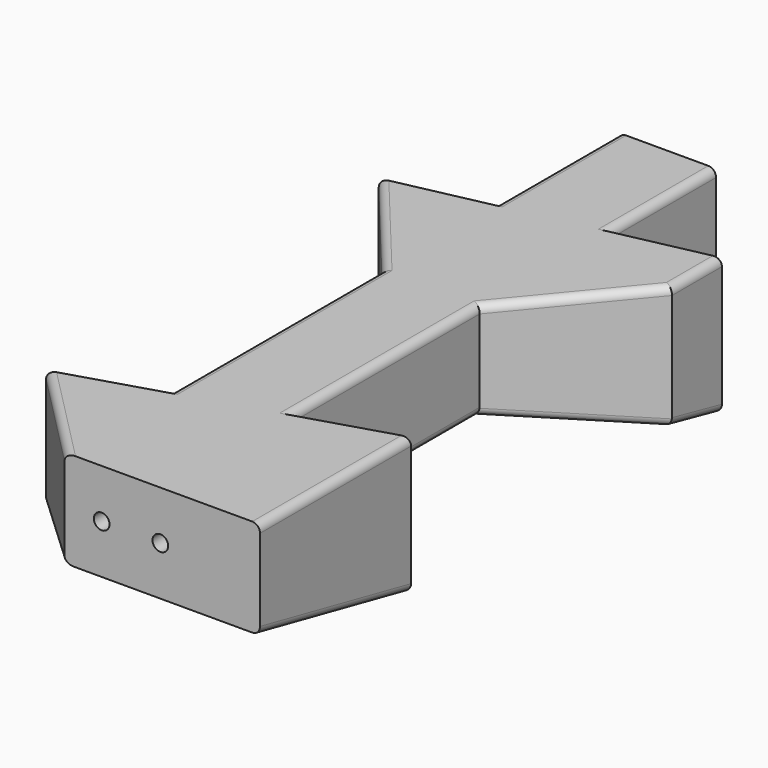
from build123d import *

# Parameters (mm, degrees)
F0_W           = 25
F0_H           = 33
F1_DEPTH       = 25
F3_DEPTH       = 10
F5_DEPTH       = 81.7
F7_DEPTH       = 10
F9_DEPTH       = 92
F10_W          = 13
F10_H          = 13
F11_DEPTH      = 135
F12_R          = 1.9
F13_DEPTH      = 7
F14_R          = 1.9
F15_DEPTH      = 7
F17_DEPTH      = 18
F18_T1_DEPTH   = 26.3114146799
F18_T3_DEPTH   = 25.9417421253
F18_T5_DEPTH   = 59.3111485648
F18_T7_DEPTH   = 58.2865340729
F18_T9_DEPTH   = 45.6084808239
F18_T11_DEPTH  = 44.6581070284
F18_T16_DEPTH  = 49.2253281189
F18_T21_DEPTH  = 48.4985768834
F18_T27_DEPTH  = 48.4985768834
F18_T33_DEPTH  = 48.4985768834
F18_T39_DEPTH  = 48.4985768834
F18_T45_DEPTH  = 48.4985768834
F18_T51_DEPTH  = 48.4985768834
F18_T57_DEPTH  = 49.2253281189
F18_T62_DEPTH  = 70.8165659944
F18_T69_DEPTH  = 70.8165659944
F18_T75_DEPTH  = 70.8165659944
F18_T81_DEPTH  = 70.8165659944
F18_T87_DEPTH  = 78.4598330308
F18_T93_DEPTH  = 78.4598330308
F18_T99_DEPTH  = 78.4598330308
F18_T106_DEPTH = 78.4598330308
F18_T112_DEPTH = 50
F18_T117_DEPTH = 50
F18_T122_DEPTH = 44.6860859582
F18_T127_DEPTH = 44.6860859582
F18_T133_DEPTH = 70.8165659944
F18_T137_DEPTH = 49.2253281189
F18_T144_DEPTH = 70.8165659944
F18_T149_DEPTH = 48.4985768834
F18_T157_DEPTH = 48.4985768834
F18_T162_DEPTH = 78.4598330308
F18_T170_DEPTH = 49.2253281189
F18_T174_DEPTH = 78.4598330308


# Not quite as in the source:
# - a fillet or chamfer that OpenCascade refuses, or shapes differently, is made with other operations: its cross-section is extruded or revolved along the edge and cut away or added


with BuildPart() as f1:
    # F0 (on Top) → F1 (new body)
    with BuildSketch(Plane.XY):
        with Locations((12.5, 16.5)):
            Rectangle(F0_W, F0_H)
        Polygon((-25, 25.3567329635), (0, 0), (0, 33), align=None)
        with Locations((37.5, 16.5)):
            Rectangle(F0_W, F0_H)
        Polygon((25, 40.6432670365), (0, 33), (25, 33), align=None)
        Polygon((0, 101.4598330308), (0, 33), (25, 40.6432670365), (25, 101.4598330308), (25, 137), (0, 137), align=None)
        Polygon((25, 40.6432670365), (25, 33), (50, 33), (50, 48.2865340729), align=None)
        Polygon((-25, 131.6860859582), (0, 101.4598330308), (0, 137), align=None)
        Polygon((25, 137), (25, 101.4598330308), (50, 131.6860859582), (50, 147.6278280835), (25, 142.3139140418), align=None)
        Polygon((25, 142.3139140418), (0, 137), (25, 137), align=None)
        Polygon((0, 177), (0, 137), (25, 142.3139140418), (25, 177), align=None)
    extrude(amount=F1_DEPTH)

    # F2 (on face) → F3 (join)
    with BuildSketch(Plane(origin=(0, 0, 0), x_dir=(1, 0, 0), z_dir=(0, 0, -1))):
        Polygon((50, -131.6860859582), (25, -101.4598330308), (0, -101.4598330308), (-25, -131.6860859582), (50, -147.6278280835), align=None)
    extrude(amount=F3_DEPTH)

    # F4 (on face) → F5 (cut, symmetric)
    with BuildSketch(Plane.YZ.offset(25)):
        Polygon((101.4598330308, -21.1370438337), (147.6278330308, -10), (101.4598330308, 0), align=None)
    extrude(amount=F5_DEPTH, both=True, mode=Mode.SUBTRACT)

    # F6 (on face) → F7 (join)
    with BuildSketch(Plane(origin=(0, 0, 0), x_dir=(1, 0, 0), z_dir=(0, 0, -1))):
        Polygon((50, -48.2865340729), (50, 0), (0, 0), (-25, -25.3567329635), align=None)
    extrude(amount=F7_DEPTH)

    # F8 (on face) → F9 (cut)
    with BuildSketch(Plane.YZ.offset(50)):
        Polygon((48.2865340729, -10), (0, 0), (0, -39.534393698), (48.2865340729, -39.534393698), align=None)
    extrude(amount=-F9_DEPTH, mode=Mode.SUBTRACT)

    # F10 (on face) → F11 (cut)
    with BuildSketch(Plane(origin=(0, 177, 0), x_dir=(-1, 0, 0), z_dir=(0, 1, 0))):
        with Locations((-12.5, 12.5)):
            Rectangle(F10_W, F10_H)
    extrude(amount=-F11_DEPTH, mode=Mode.SUBTRACT)

    # F12 (on face) → F13 (cut)
    with BuildSketch(Plane(origin=(-27.8614600507, 131.0778638485, 0), x_dir=(-0.9781476007, -0.2079116908, 0), z_dir=(-0.2079116908, 0.9781476007, 0))):
        with Locations((-18.6253867704, 12.5)):
            Circle(F12_R)
        with BuildLine():
            ThreePointArc((-72.2009313853, 12.5), (-70.3009313853, 10.6), (-68.4009313853, 12.5))
            ThreePointArc((-68.4009313853, 12.5), (-70.3009313853, 14.4), (-72.2009313853, 12.5))
        make_face()
    extrude(amount=-F13_DEPTH, mode=Mode.SUBTRACT)

    # F14 (on face) → F15 (cut)
    with BuildSketch(Plane(origin=(-9.2266829073, 30.1791199472, 0), x_dir=(-0.956304756, -0.2923717047, 0), z_dir=(-0.2923717047, 0.956304756, 0))):
        with Locations((0.6940276563, 12.5)):
            Circle(F14_R)
        with BuildLine():
            ThreePointArc((-54.6362143833, 12.2785296088), (-52.7659137894, 10.3211052927), (-50.8370889828, 12.2208866302))
            ThreePointArc((-50.8370889828, 12.2208866302), (-52.7082641762, 14.1206679678), (-54.6362143833, 12.2785296088))
        make_face()
    extrude(amount=-F15_DEPTH, mode=Mode.SUBTRACT)

    # F16 (on face) → F17 (cut)
    with BuildSketch(Plane.XZ):
        with BuildLine():
            ThreePointArc((11.5, 12.5), (9.5, 14.5), (7.5, 12.5))
            Line((7.5, 12.5), (9.5, 12.5))
            Line((9.5, 12.5), (11.5, 12.5))
        make_face()
        with BuildLine():
            ThreePointArc((26.5, 12.5), (24.5, 14.5), (22.5, 12.5))
            ThreePointArc((22.5, 12.5), (24.5, 10.5), (26.5, 12.5))
        make_face()
        with BuildLine():
            Line((9.5, 12.5), (7.5, 12.5))
            ThreePointArc((7.5, 12.5), (9.5, 10.5), (11.5, 12.5))
            Line((11.5, 12.5), (9.5, 12.5))
        make_face()
    extrude(amount=-F17_DEPTH, mode=Mode.SUBTRACT)

    # F18: fillet of radius 2 on 18 edges, made by hand

    # F18_s2 → F18_t1 (cut)
    with BuildSketch(Plane(origin=(0, 122.2526609766, -26.4799560251), x_dir=(1, 0, 0), z_dir=(0, 0.9773365731, -0.2116913388))):
        with BuildLine():
            ThreePointArc((50, -23.478167891), (49.4142135624, -22.0639543286), (48, -21.478167891))
            Line((48, -21.478167891), (50, -21.478167891))
            Line((50, -21.478167891), (50, -23.478167891))
        make_face()
    extrude(amount=F18_T1_DEPTH, mode=Mode.SUBTRACT)

    # F18_s4 → F18_t3 (cut)
    with BuildSketch(Plane.XZ.offset(-152.6278280835)):
        with BuildLine():
            ThreePointArc((48, 25), (49.4142135624, 24.4142135624), (50, 23))
            Line((50, 23), (50, 25))
            Line((50, 25), (48, 25))
        make_face()
    extrude(amount=F18_T3_DEPTH, mode=Mode.SUBTRACT)

    # F18_s6 → F18_t5 (cut)
    with BuildSketch(Plane(origin=(0, 53.1826412899, -11.0139694867), x_dir=(1, 0, 0), z_dir=(0, -0.9792214434, 0.2027938973))):
        with BuildLine():
            ThreePointArc((48, 0), (49.4142135624, 0.5857864376), (50, 2))
            Line((50, 2), (50, 0))
            Line((50, 0), (48, 0))
        make_face()
    extrude(amount=F18_T5_DEPTH, mode=Mode.SUBTRACT)

    # F18_s8 → F18_t7 (cut)
    with BuildSketch(Plane.XZ.offset(-53.2865340729)):
        with BuildLine():
            ThreePointArc((48, 25), (49.4142135624, 24.4142135624), (50, 23))
            Line((50, 23), (50, 25))
            Line((50, 25), (48, 25))
        make_face()
    extrude(amount=F18_T7_DEPTH, mode=Mode.SUBTRACT)

    # F18_s10 → F18_t9 (cut)
    with BuildSketch(Plane(origin=(-28.5103996887, 28.9172236636, 0), x_dir=(0, 0, 1), z_dir=(0.7020799377, -0.71209814, 0))):
        with BuildLine():
            ThreePointArc((23, 0), (24.4142135624, -0.5857864376), (25, -2))
            Line((25, -2), (25, 0))
            Line((25, 0), (23, 0))
        make_face()
    extrude(amount=F18_T9_DEPTH, mode=Mode.SUBTRACT)

    # F18_s12 → F18_t11 (cut)
    with BuildSketch(Plane(origin=(-28.0090391043, 28.4087090053, -5.8833605581), x_dir=(0.71209814, 0.7020799377, 0), z_dir=(0.6945676893, -0.7044786969, 0.145895478))):
        with BuildLine():
            ThreePointArc((0, 1.7328989819), (0.4884593774, 0.4232253789), (1.7152449464, -0.2467258713))
            Line((1.7152449464, -0.2467258713), (0, 0))
            Line((0, 0), (0, 1.7328989819))
        make_face()
    extrude(amount=F18_T11_DEPTH, mode=Mode.SUBTRACT)


with BuildPart() as f18_tool14:
    # F18_s15 → F18_t16 (new body)
    with BuildSketch(Plane(origin=(56.7978037382, 68.6713912604, 0), x_dir=(0, 0, 1), z_dir=(0.6373432983, 0.7705799894, 0))):
        with BuildLine():
            ThreePointArc((25, -47.4002448925), (24.4142135624, -45.9860313302), (23, -45.4002448925))
            Line((23, -45.4002448925), (25, -45.4002448925))
            Line((25, -45.4002448925), (25, -47.4002448925))
        make_face()
    extrude(amount=F18_T16_DEPTH)

    split(bisect_by=Plane.YZ.offset(25), keep=Keep.TOP)


with BuildPart() as f1_1:
    add(f1.part)

    # F18_t13: cut F18_tool14
    add(f18_tool14.part, mode=Mode.SUBTRACT)


with BuildPart() as f18_tool19:
    # F18_s20 → F18_t21 (new body)
    with BuildSketch(Plane(origin=(55.6145080943, 67.2407275237, -14.5643578937), x_dir=(-0.7705799894, 0.6373432983, 0), z_dir=(0.6286469564, 0.7600656763, -0.1646304099))):
        with BuildLine():
            ThreePointArc((45.4002448925, 17.2405635017), (45.8936460368, 15.9252080791), (47.1304047803, 15.258850527))
            Line((47.1304047803, 15.258850527), (45.4002448925, 15.4944378922))
            Line((45.4002448925, 15.4944378922), (45.4002448925, 17.2405635017))
        make_face()
    extrude(amount=F18_T21_DEPTH)

    split(bisect_by=Plane.YZ.offset(25), keep=Keep.BOTTOM)

    split(bisect_by=Plane.XY, keep=Keep.BOTTOM)


with BuildPart() as f1_2:
    add(f1_1.part)

    # F18_t18: cut F18_tool19
    add(f18_tool19.part, mode=Mode.SUBTRACT)


with BuildPart() as f18_tool25:
    # F18_s26 → F18_t27 (new body)
    with BuildSketch(Plane(origin=(55.6145080943, 67.2407275237, -14.5643578937), x_dir=(-0.7705799894, 0.6373432983, 0), z_dir=(0.6286469564, 0.7600656763, -0.1646304099))):
        with BuildLine():
            ThreePointArc((45.4002448925, 17.2405635017), (45.8936460368, 15.9252080791), (47.1304047803, 15.258850527))
            Line((47.1304047803, 15.258850527), (45.4002448925, 15.4944378922))
            Line((45.4002448925, 15.4944378922), (45.4002448925, 17.2405635017))
        make_face()
    extrude(amount=F18_T27_DEPTH)

    split(bisect_by=Plane.YZ.offset(25), keep=Keep.TOP)

    split(bisect_by=Plane.XY, keep=Keep.TOP)


with BuildPart() as f1_3:
    add(f1_2.part)

    # F18_t24: cut F18_tool25
    add(f18_tool25.part, mode=Mode.SUBTRACT)


with BuildPart() as f18_tool31:
    # F18_s32 → F18_t33 (new body)
    with BuildSketch(Plane(origin=(55.6145080943, 67.2407275237, -14.5643578937), x_dir=(-0.7705799894, 0.6373432983, 0), z_dir=(0.6286469564, 0.7600656763, -0.1646304099))):
        with BuildLine():
            ThreePointArc((45.4002448925, 17.2405635017), (45.8936460368, 15.9252080791), (47.1304047803, 15.258850527))
            Line((47.1304047803, 15.258850527), (45.4002448925, 15.4944378922))
            Line((45.4002448925, 15.4944378922), (45.4002448925, 17.2405635017))
        make_face()
    extrude(amount=F18_T33_DEPTH)

    split(bisect_by=Plane.YZ.offset(25), keep=Keep.TOP)

    split(bisect_by=Plane.XY, keep=Keep.BOTTOM)


with BuildPart() as f1_4:
    add(f1_3.part)

    # F18_t30: cut F18_tool31
    add(f18_tool31.part, mode=Mode.SUBTRACT)


with BuildPart() as f18_tool37:
    # F18_s38 → F18_t39 (new body)
    with BuildSketch(Plane(origin=(-76.2230659478, 92.1575068097, -19.9613383317), x_dir=(0.7705799894, 0.6373432983, 0), z_dir=(0.6286469564, -0.7600656763, 0.1646304099))):
        with BuildLine():
            ThreePointArc((64.6647446284, 14.617411291), (65.1581457726, 13.3020558683), (66.3949045162, 12.6356983163))
            Line((66.3949045162, 12.6356983163), (64.6647446284, 12.8712856815))
            Line((64.6647446284, 12.8712856815), (64.6647446284, 14.617411291))
        make_face()
    extrude(amount=F18_T39_DEPTH)

    split(bisect_by=Plane.YZ, keep=Keep.BOTTOM)

    split(bisect_by=Plane.XY, keep=Keep.BOTTOM)


with BuildPart() as f1_5:
    add(f1_4.part)

    # F18_t36: cut F18_tool37
    add(f18_tool37.part, mode=Mode.SUBTRACT)


with BuildPart() as f18_tool43:
    # F18_s44 → F18_t45 (new body)
    with BuildSketch(Plane(origin=(-76.2230659478, 92.1575068097, -19.9613383317), x_dir=(0.7705799894, 0.6373432983, 0), z_dir=(0.6286469564, -0.7600656763, 0.1646304099))):
        with BuildLine():
            ThreePointArc((64.6647446284, 14.617411291), (65.1581457726, 13.3020558683), (66.3949045162, 12.6356983163))
            Line((66.3949045162, 12.6356983163), (64.6647446284, 12.8712856815))
            Line((64.6647446284, 12.8712856815), (64.6647446284, 14.617411291))
        make_face()
    extrude(amount=F18_T45_DEPTH)

    split(bisect_by=Plane.YZ, keep=Keep.TOP)

    split(bisect_by=Plane.XY, keep=Keep.BOTTOM)


with BuildPart() as f1_6:
    add(f1_5.part)

    # F18_t42: cut F18_tool43
    add(f18_tool43.part, mode=Mode.SUBTRACT)


with BuildPart() as f18_tool49:
    # F18_s50 → F18_t51 (new body)
    with BuildSketch(Plane(origin=(-76.2230659478, 92.1575068097, -19.9613383317), x_dir=(0.7705799894, 0.6373432983, 0), z_dir=(0.6286469564, -0.7600656763, 0.1646304099))):
        with BuildLine():
            ThreePointArc((64.6647446284, 14.617411291), (65.1581457726, 13.3020558683), (66.3949045162, 12.6356983163))
            Line((66.3949045162, 12.6356983163), (64.6647446284, 12.8712856815))
            Line((64.6647446284, 12.8712856815), (64.6647446284, 14.617411291))
        make_face()
    extrude(amount=F18_T51_DEPTH)

    split(bisect_by=Plane.YZ, keep=Keep.BOTTOM)

    split(bisect_by=Plane.XY, keep=Keep.TOP)


with BuildPart() as f1_7:
    add(f1_6.part)

    # F18_t48: cut F18_tool49
    add(f18_tool49.part, mode=Mode.SUBTRACT)


with BuildPart() as f18_tool55:
    # F18_s56 → F18_t57 (new body)
    with BuildSketch(Plane(origin=(-78.016074724, 94.3253442805, 0), x_dir=(0, 0, 1), z_dir=(0.6373432983, -0.7705799894, 0))):
        with BuildLine():
            ThreePointArc((25, -66.6647446284), (24.4142135624, -65.250531066), (23, -64.6647446284))
            Line((23, -64.6647446284), (25, -64.6647446284))
            Line((25, -64.6647446284), (25, -66.6647446284))
        make_face()
    extrude(amount=F18_T57_DEPTH)

    split(bisect_by=Plane.YZ, keep=Keep.BOTTOM)


with BuildPart() as f1_8:
    add(f1_7.part)

    # F18_t54: cut F18_tool55
    add(f18_tool55.part, mode=Mode.SUBTRACT)


with BuildPart() as f18_tool60:
    # F18_s61 → F18_t62 (new body)
    with BuildSketch(Plane.XZ.offset(-35.6432670365)):
        with BuildLine():
            ThreePointArc((25, 2), (24.4142135624, 0.5857864376), (23, 0))
            Line((23, 0), (25, 0))
            Line((25, 0), (25, 2))
        make_face()
    extrude(amount=-F18_T62_DEPTH)

    split(bisect_by=Plane(origin=(-9.2266829073, 30.1791199472, 0), x_dir=(0, 0, 1), z_dir=(-0.2923717047, 0.956304756, 0)), keep=Keep.TOP)

    split(bisect_by=Plane(origin=(-34.9845202296, 28.9355418232, 0), x_dir=(0, 0, 1), z_dir=(0.7705799894, -0.6373432983, 0)), keep=Keep.TOP)

    split(bisect_by=Plane(origin=(0, 4.5467421163, 20.9913990025), x_dir=(1, 0, 0), z_dir=(0, -0.2116913388, -0.9773365731)), keep=Keep.TOP)


with BuildPart() as f1_9:
    add(f1_8.part)

    # F18_t59: cut F18_tool60
    add(f18_tool60.part, mode=Mode.SUBTRACT)


with BuildPart() as f18_tool67:
    # F18_s68 → F18_t69 (new body)
    with BuildSketch(Plane.XZ.offset(-35.6432670365)):
        with BuildLine():
            ThreePointArc((25, 2), (24.4142135624, 0.5857864376), (23, 0))
            Line((23, 0), (25, 0))
            Line((25, 0), (25, 2))
        make_face()
    extrude(amount=-F18_T69_DEPTH)

    split(bisect_by=Plane(origin=(-34.9845202296, 28.9355418232, 0), x_dir=(0, 0, 1), z_dir=(-0.7705799894, 0.6373432983, 0)), keep=Keep.TOP)

    split(bisect_by=Plane(origin=(0, 4.5467421163, 20.9913990025), x_dir=(1, 0, 0), z_dir=(0, -0.2116913388, -0.9773365731)), keep=Keep.TOP)


with BuildPart() as f1_10:
    add(f1_9.part)

    # F18_t66: cut F18_tool67
    add(f18_tool67.part, mode=Mode.SUBTRACT)


with BuildPart() as f18_tool73:
    # F18_s74 → F18_t75 (new body)
    with BuildSketch(Plane.XZ.offset(-35.6432670365)):
        with BuildLine():
            ThreePointArc((25, 2), (24.4142135624, 0.5857864376), (23, 0))
            Line((23, 0), (25, 0))
            Line((25, 0), (25, 2))
        make_face()
    extrude(amount=-F18_T75_DEPTH)

    split(bisect_by=Plane(origin=(-34.9845202296, 28.9355418232, 0), x_dir=(0, 0, 1), z_dir=(0.7705799894, -0.6373432983, 0)), keep=Keep.TOP)

    split(bisect_by=Plane(origin=(0, 4.5467421163, 20.9913990025), x_dir=(1, 0, 0), z_dir=(0, 0.2116913388, 0.9773365731)), keep=Keep.TOP)


with BuildPart() as f1_11:
    add(f1_10.part)

    # F18_t72: cut F18_tool73
    add(f18_tool73.part, mode=Mode.SUBTRACT)


with BuildPart() as f18_tool79:
    # F18_s80 → F18_t81 (new body)
    with BuildSketch(Plane.XZ.offset(-35.6432670365)):
        with BuildLine():
            ThreePointArc((23, 25), (24.4142135624, 24.4142135624), (25, 23))
            Line((25, 23), (25, 25))
            Line((25, 25), (23, 25))
        make_face()
    extrude(amount=-F18_T81_DEPTH)

    split(bisect_by=Plane(origin=(-9.2266829073, 30.1791199472, 0), x_dir=(0, 0, 1), z_dir=(-0.2923717047, 0.956304756, 0)), keep=Keep.TOP)

    split(bisect_by=Plane(origin=(-34.9845202296, 28.9355418232, 0), x_dir=(0, 0, 1), z_dir=(0.7705799894, -0.6373432983, 0)), keep=Keep.TOP)


with BuildPart() as f1_12:
    add(f1_11.part)

    # F18_t78: cut F18_tool79
    add(f18_tool79.part, mode=Mode.SUBTRACT)


with BuildPart() as f18_tool85:
    # F18_s86 → F18_t87 (new body)
    with BuildSketch(Plane.XZ.offset(-106.4598330308)):
        with BuildLine():
            ThreePointArc((0, 2), (0.5857864376, 0.5857864376), (2, 0))
            Line((2, 0), (0, 0))
            Line((0, 0), (0, 2))
        make_face()
    extrude(amount=F18_T87_DEPTH)

    split(bisect_by=Plane(origin=(49.8293582326, 41.2136416249, 0), x_dir=(0, 0, 1), z_dir=(0.7705799894, 0.6373432983, 0)), keep=Keep.TOP)

    split(bisect_by=Plane(origin=(0, 4.5467421163, 20.9913990025), x_dir=(1, 0, 0), z_dir=(0, -0.2116913388, -0.9773365731)), keep=Keep.TOP)


with BuildPart() as f1_13:
    add(f1_12.part)

    # F18_t84: cut F18_tool85
    add(f18_tool85.part, mode=Mode.SUBTRACT)


with BuildPart() as f18_tool91:
    # F18_s92 → F18_t93 (new body)
    with BuildSketch(Plane.XZ.offset(-106.4598330308)):
        with BuildLine():
            ThreePointArc((0, 2), (0.5857864376, 0.5857864376), (2, 0))
            Line((2, 0), (0, 0))
            Line((0, 0), (0, 2))
        make_face()
    extrude(amount=F18_T93_DEPTH)

    split(bisect_by=Plane(origin=(49.8293582326, 41.2136416249, 0), x_dir=(0, 0, 1), z_dir=(-0.7705799894, -0.6373432983, 0)), keep=Keep.TOP)

    split(bisect_by=Plane(origin=(0, 4.5467421163, 20.9913990025), x_dir=(1, 0, 0), z_dir=(0, 0.2116913388, 0.9773365731)), keep=Keep.TOP)


with BuildPart() as f1_14:
    add(f1_13.part)

    # F18_t90: cut F18_tool91
    add(f18_tool91.part, mode=Mode.SUBTRACT)


with BuildPart() as f18_tool97:
    # F18_s98 → F18_t99 (new body)
    with BuildSketch(Plane.XZ.offset(-106.4598330308)):
        with BuildLine():
            ThreePointArc((0, 2), (0.5857864376, 0.5857864376), (2, 0))
            Line((2, 0), (0, 0))
            Line((0, 0), (0, 2))
        make_face()
    extrude(amount=F18_T99_DEPTH)

    split(bisect_by=Plane(origin=(-9.2266829073, 30.1791199472, 0), x_dir=(0, 0, 1), z_dir=(-0.2923717047, 0.956304756, 0)), keep=Keep.TOP)

    split(bisect_by=Plane(origin=(49.8293582326, 41.2136416249, 0), x_dir=(0, 0, 1), z_dir=(-0.7705799894, -0.6373432983, 0)), keep=Keep.TOP)

    split(bisect_by=Plane(origin=(0, 4.5467421163, 20.9913990025), x_dir=(1, 0, 0), z_dir=(0, -0.2116913388, -0.9773365731)), keep=Keep.TOP)


with BuildPart() as f1_15:
    add(f1_14.part)

    # F18_t96: cut F18_tool97
    add(f18_tool97.part, mode=Mode.SUBTRACT)


with BuildPart() as f18_tool104:
    # F18_s105 → F18_t106 (new body)
    with BuildSketch(Plane.XZ.offset(-106.4598330308)):
        with BuildLine():
            ThreePointArc((2, 25), (0.5857864376, 24.4142135624), (0, 23))
            Line((0, 23), (0, 25))
            Line((0, 25), (2, 25))
        make_face()
    extrude(amount=F18_T106_DEPTH)

    split(bisect_by=Plane(origin=(-9.2266829073, 30.1791199472, 0), x_dir=(0, 0, 1), z_dir=(-0.2923717047, 0.956304756, 0)), keep=Keep.TOP)

    split(bisect_by=Plane(origin=(49.8293582326, 41.2136416249, 0), x_dir=(0, 0, 1), z_dir=(-0.7705799894, -0.6373432983, 0)), keep=Keep.TOP)


with BuildPart() as f1_16:
    add(f1_15.part)

    # F18_t103: cut F18_tool104
    add(f18_tool104.part, mode=Mode.SUBTRACT)


with BuildPart() as f18_tool110:
    # F18_s111 → F18_t112 (new body)
    with BuildSketch(Plane.XZ.offset(-182)):
        with BuildLine():
            ThreePointArc((0, 2), (0.5857864376, 0.5857864376), (2, 0))
            Line((2, 0), (0, 0))
            Line((0, 0), (0, 2))
        make_face()
    extrude(amount=F18_T112_DEPTH)

    split(bisect_by=Plane(origin=(-27.8614600507, 131.0778638485, 0), x_dir=(0, 0, 1), z_dir=(-0.2079116908, 0.9781476007, 0)), keep=Keep.TOP)


with BuildPart() as f1_17:
    add(f1_16.part)

    # F18_t109: cut F18_tool110
    add(f18_tool110.part, mode=Mode.SUBTRACT)


with BuildPart() as f18_tool115:
    # F18_s116 → F18_t117 (new body)
    with BuildSketch(Plane.XZ.offset(-182)):
        with BuildLine():
            ThreePointArc((2, 25), (0.5857864376, 24.4142135624), (0, 23))
            Line((0, 23), (0, 25))
            Line((0, 25), (2, 25))
        make_face()
    extrude(amount=F18_T117_DEPTH)

    split(bisect_by=Plane(origin=(-27.8614600507, 131.0778638485, 0), x_dir=(0, 0, 1), z_dir=(-0.2079116908, 0.9781476007, 0)), keep=Keep.TOP)


with BuildPart() as f1_18:
    add(f1_17.part)

    # F18_t114: cut F18_tool115
    add(f18_tool115.part, mode=Mode.SUBTRACT)


with BuildPart() as f18_tool120:
    # F18_s121 → F18_t122 (new body)
    with BuildSketch(Plane.XZ.offset(-137.3139140418)):
        with BuildLine():
            ThreePointArc((23, 25), (24.4142135624, 24.4142135624), (25, 23))
            Line((25, 23), (25, 25))
            Line((25, 25), (23, 25))
        make_face()
    extrude(amount=-F18_T122_DEPTH)

    split(bisect_by=Plane(origin=(-27.8614600507, 131.0778638485, 0), x_dir=(0, 0, 1), z_dir=(-0.2079116908, 0.9781476007, 0)), keep=Keep.TOP)


with BuildPart() as f1_19:
    add(f1_18.part)

    # F18_t119: cut F18_tool120
    add(f18_tool120.part, mode=Mode.SUBTRACT)


with BuildPart() as f18_tool125:
    # F18_s126 → F18_t127 (new body)
    with BuildSketch(Plane.XZ.offset(-137.3139140418)):
        with BuildLine():
            ThreePointArc((25, 2), (24.4142135624, 0.5857864376), (23, 0))
            Line((23, 0), (25, 0))
            Line((25, 0), (25, 2))
        make_face()
    extrude(amount=-F18_T127_DEPTH)

    split(bisect_by=Plane(origin=(-27.8614600507, 131.0778638485, 0), x_dir=(0, 0, 1), z_dir=(-0.2079116908, 0.9781476007, 0)), keep=Keep.TOP)


with BuildPart() as f1_20:
    add(f1_19.part)

    # F18_t124: cut F18_tool125
    add(f18_tool125.part, mode=Mode.SUBTRACT)


with BuildPart() as f18_tool131:
    # F18_s132 → F18_t133 (new body)
    with BuildSketch(Plane.XZ.offset(-35.6432670365)):
        with BuildLine():
            ThreePointArc((23, 25), (24.4142135624, 24.4142135624), (25, 23))
            Line((25, 23), (25, 25))
            Line((25, 25), (23, 25))
        make_face()
    extrude(amount=-F18_T133_DEPTH)

    split(bisect_by=Plane(origin=(-34.9845202296, 28.9355418232, 0), x_dir=(0, 0, 1), z_dir=(-0.7705799894, 0.6373432983, 0)), keep=Keep.TOP)


with BuildPart() as f18_tool135:
    # F18_s136 → F18_t137 (new body)
    with BuildSketch(Plane(origin=(56.7978037382, 68.6713912604, 0), x_dir=(0, 0, 1), z_dir=(0.6373432983, 0.7705799894, 0))):
        with BuildLine():
            ThreePointArc((25, -47.4002448925), (24.4142135624, -45.9860313302), (23, -45.4002448925))
            Line((23, -45.4002448925), (25, -45.4002448925))
            Line((25, -45.4002448925), (25, -47.4002448925))
        make_face()
    extrude(amount=F18_T137_DEPTH)

    split(bisect_by=Plane.YZ.offset(25), keep=Keep.BOTTOM)


with BuildPart() as f18_tool131_1:
    add(f18_tool131.part)

    # F18_t139: intersect F18_tool135
    add(f18_tool135.part, mode=Mode.INTERSECT)


with BuildPart() as f1_21:
    add(f1_20.part)

    # F18_t129: cut F18_tool131
    add(f18_tool131_1.part, mode=Mode.SUBTRACT)


with BuildPart() as f18_tool142:
    # F18_s143 → F18_t144 (new body)
    with BuildSketch(Plane.XZ.offset(-35.6432670365)):
        with BuildLine():
            ThreePointArc((25, 2), (24.4142135624, 0.5857864376), (23, 0))
            Line((23, 0), (25, 0))
            Line((25, 0), (25, 2))
        make_face()
    extrude(amount=-F18_T144_DEPTH)

    split(bisect_by=Plane(origin=(-34.9845202296, 28.9355418232, 0), x_dir=(0, 0, 1), z_dir=(-0.7705799894, 0.6373432983, 0)), keep=Keep.TOP)

    split(bisect_by=Plane(origin=(0, 4.5467421163, 20.9913990025), x_dir=(1, 0, 0), z_dir=(0, 0.2116913388, 0.9773365731)), keep=Keep.TOP)


with BuildPart() as f18_tool147:
    # F18_s148 → F18_t149 (new body)
    with BuildSketch(Plane(origin=(55.6145080943, 67.2407275237, -14.5643578937), x_dir=(-0.7705799894, 0.6373432983, 0), z_dir=(0.6286469564, 0.7600656763, -0.1646304099))):
        with BuildLine():
            ThreePointArc((45.4002448925, 17.2405635017), (45.8936460368, 15.9252080791), (47.1304047803, 15.258850527))
            Line((47.1304047803, 15.258850527), (45.4002448925, 15.4944378922))
            Line((45.4002448925, 15.4944378922), (45.4002448925, 17.2405635017))
        make_face()
    extrude(amount=F18_T149_DEPTH)

    split(bisect_by=Plane.YZ.offset(25), keep=Keep.BOTTOM)

    split(bisect_by=Plane.XY, keep=Keep.TOP)


with BuildPart() as f18_tool142_1:
    add(f18_tool142.part)

    # F18_t152: intersect F18_tool147
    add(f18_tool147.part, mode=Mode.INTERSECT)


with BuildPart() as f1_22:
    add(f1_21.part)

    # F18_t140: cut F18_tool142
    add(f18_tool142_1.part, mode=Mode.SUBTRACT)


with BuildPart() as f18_tool155:
    # F18_s156 → F18_t157 (new body)
    with BuildSketch(Plane(origin=(-76.2230659478, 92.1575068097, -19.9613383317), x_dir=(0.7705799894, 0.6373432983, 0), z_dir=(0.6286469564, -0.7600656763, 0.1646304099))):
        with BuildLine():
            ThreePointArc((64.6647446284, 14.617411291), (65.1581457726, 13.3020558683), (66.3949045162, 12.6356983163))
            Line((66.3949045162, 12.6356983163), (64.6647446284, 12.8712856815))
            Line((64.6647446284, 12.8712856815), (64.6647446284, 14.617411291))
        make_face()
    extrude(amount=F18_T157_DEPTH)

    split(bisect_by=Plane.YZ, keep=Keep.TOP)

    split(bisect_by=Plane.XY, keep=Keep.TOP)


with BuildPart() as f18_tool160:
    # F18_s161 → F18_t162 (new body)
    with BuildSketch(Plane.XZ.offset(-106.4598330308)):
        with BuildLine():
            ThreePointArc((0, 2), (0.5857864376, 0.5857864376), (2, 0))
            Line((2, 0), (0, 0))
            Line((0, 0), (0, 2))
        make_face()
    extrude(amount=F18_T162_DEPTH)

    split(bisect_by=Plane(origin=(49.8293582326, 41.2136416249, 0), x_dir=(0, 0, 1), z_dir=(0.7705799894, 0.6373432983, 0)), keep=Keep.TOP)

    split(bisect_by=Plane(origin=(0, 4.5467421163, 20.9913990025), x_dir=(1, 0, 0), z_dir=(0, 0.2116913388, 0.9773365731)), keep=Keep.TOP)


with BuildPart() as f18_tool155_1:
    add(f18_tool155.part)

    # F18_t165: intersect F18_tool160
    add(f18_tool160.part, mode=Mode.INTERSECT)


with BuildPart() as f1_23:
    add(f1_22.part)

    # F18_t153: cut F18_tool155
    add(f18_tool155_1.part, mode=Mode.SUBTRACT)


with BuildPart() as f18_tool168:
    # F18_s169 → F18_t170 (new body)
    with BuildSketch(Plane(origin=(-78.016074724, 94.3253442805, 0), x_dir=(0, 0, 1), z_dir=(0.6373432983, -0.7705799894, 0))):
        with BuildLine():
            ThreePointArc((25, -66.6647446284), (24.4142135624, -65.250531066), (23, -64.6647446284))
            Line((23, -64.6647446284), (25, -64.6647446284))
            Line((25, -64.6647446284), (25, -66.6647446284))
        make_face()
    extrude(amount=F18_T170_DEPTH)

    split(bisect_by=Plane.YZ, keep=Keep.TOP)


with BuildPart() as f18_tool172:
    # F18_s173 → F18_t174 (new body)
    with BuildSketch(Plane.XZ.offset(-106.4598330308)):
        with BuildLine():
            ThreePointArc((2, 25), (0.5857864376, 24.4142135624), (0, 23))
            Line((0, 23), (0, 25))
            Line((0, 25), (2, 25))
        make_face()
    extrude(amount=F18_T174_DEPTH)

    split(bisect_by=Plane(origin=(49.8293582326, 41.2136416249, 0), x_dir=(0, 0, 1), z_dir=(0.7705799894, 0.6373432983, 0)), keep=Keep.TOP)


with BuildPart() as f18_tool168_1:
    add(f18_tool168.part)

    # F18_t176: intersect F18_tool172
    add(f18_tool172.part, mode=Mode.INTERSECT)


with BuildPart() as f1_24:
    add(f1_23.part)

    # F18_t166: cut F18_tool168
    add(f18_tool168_1.part, mode=Mode.SUBTRACT)


solid = f1_24.part
